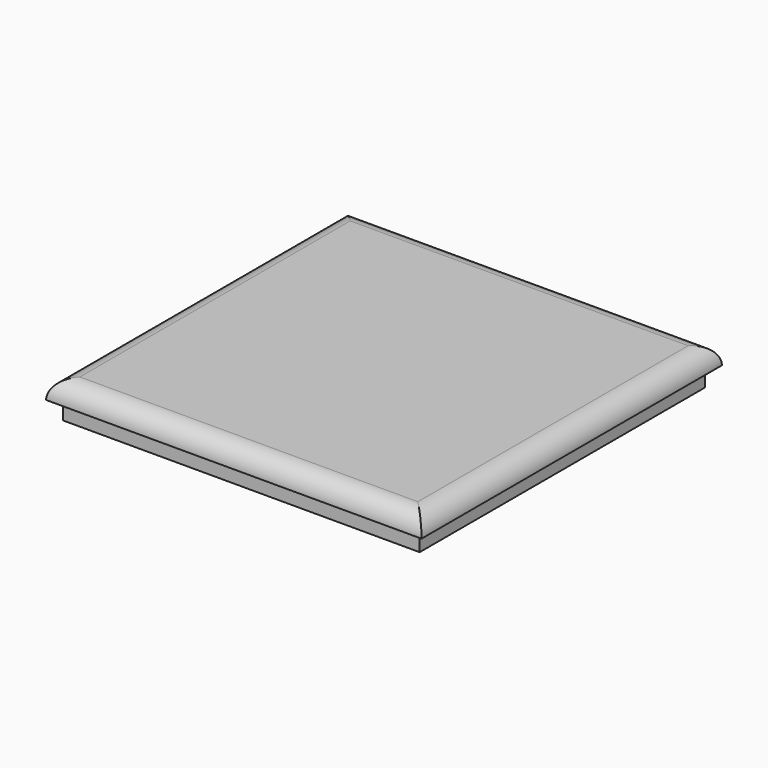
from build123d import *

# Parameters (mm, degrees)
F0_W     = 101.6
F0_H     = 101.6
F0_W_2   = 96.52
F0_H_2   = 96.52
F1_DEPTH = 5.08
F2_R     = 5.07999
F3_DEPTH = 5.08
F4_W     = 90.17
F4_H     = 90.17
F5_DEPTH = 7.62


# Not quite as in the source:
# - a fillet or chamfer is up to 0.001 mm smaller than in the source, because OpenCascade refuses the exact size


with BuildPart() as f1:
    # F0 (on Top) → F1 (new body)
    with BuildSketch(Plane.XY):
        with Locations((-46.2021417916, 16.1945652217)):
            Rectangle(F0_W, F0_H)
        with Locations((-46.2021417916, 16.1945652217)):
            Rectangle(F0_W_2, F0_H_2, mode=Mode.SUBTRACT)
        with Locations((-46.2021417916, 16.1945652217)):
            Rectangle(F0_W_2, F0_H_2)
    extrude(amount=F1_DEPTH)

    # F2 (radius 5.08 in the source; OpenCascade refuses exactly that, so slightly less here)
    f2_edges = [f1.edges().sort_by_distance(p)[0] for p in [
        (-97.002142, 16.194565, 5.08),
        (-46.202142, -34.605435, 5.08),
        (4.597858, 16.194565, 5.08),
        (-46.202142, 66.994565, 5.08),
    ]]
    fillet(f2_edges, radius=F2_R)

    # F0 (on Top) → F3 (join)
    with BuildSketch(Plane.XY):
        with Locations((-46.2021417916, 16.1945652217)):
            Rectangle(F0_W_2, F0_H_2)
    extrude(amount=-F3_DEPTH)

    # F4 (on face) → F5 (cut)
    with BuildSketch(Plane(origin=(0, 0, -5.08), x_dir=(1, 0, 0), z_dir=(0, 0, -1))):
        with Locations((-46.2021417916, -16.1945652217)):
            Rectangle(F4_W, F4_H)
    extrude(amount=-F5_DEPTH, mode=Mode.SUBTRACT)


solid = f1.part
